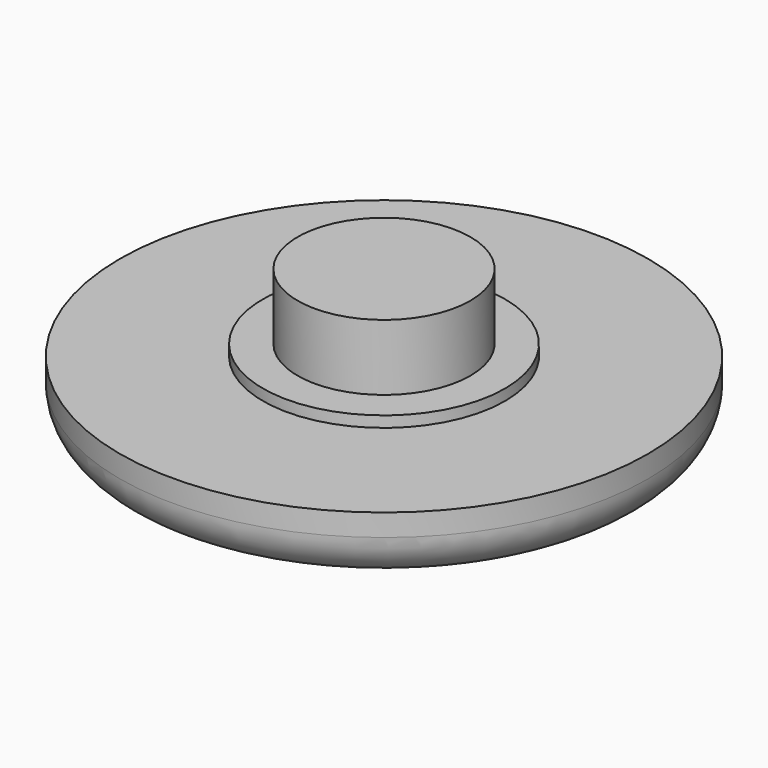
from build123d import *

# Parameters (mm, degrees)
F0_R     = 12
F1_DEPTH = 2
F2_R     = 12
F2_R_2   = 10
F3_DEPTH = 1
F4_R     = 1.99999
F5_R     = 5.5
F6_DEPTH = 0.5
F7_R     = 3.925
F8_DEPTH = 3


# Not quite as in the source:
# - a fillet or chamfer is up to 0.001 mm smaller than in the source, because OpenCascade refuses the exact size


with BuildPart() as f1:
    # F0 (on Top) → F1 (new body)
    with BuildSketch(Plane.XY):
        Circle(F0_R)
    extrude(amount=F1_DEPTH)

    # F2 (on face) → F3 (join)
    with BuildSketch(Plane(origin=(0, 0, 0), x_dir=(1, 0, 0), z_dir=(0, 0, -1))):
        Circle(F2_R)
        Circle(F2_R_2, mode=Mode.SUBTRACT)
    extrude(amount=F3_DEPTH)

    # F4 (radius 2 in the source; OpenCascade refuses exactly that, so slightly less here)
    f4_edges = [f1.edges().sort_by_distance(p)[0] for p in [
        (-12, 0, -1),
    ]]
    fillet(f4_edges, radius=F4_R)

    # F5 (on face) → F6 (join)
    with BuildSketch(Plane.XY.offset(2)):
        Circle(F5_R)
    extrude(amount=F6_DEPTH)

    # F7 (on face) → F8 (join)
    with BuildSketch(Plane.XY.offset(2.5)):
        Circle(F7_R)
    extrude(amount=F8_DEPTH)

    # F9 (on Front) → F10 (revolve)
    with BuildSketch(Plane.XZ):
        Polygon((-10.0021678954, 0), (-10.0021678954, -1.0005384684), (-9.6580199897, -0.9450307698), (-9.385343641, -0.8195927949), (-9.0745007619, -0.6752727786), (-8.19747895, -0.5198512226), (-6.5711033531, -0.3644296667), (-3.5958907101, -0.2090081107), (0, -0.0646880944), (0, 0), align=None)
    revolve(axis=Axis((0, 0, -0.0323440472), (0, 0, 1)))


solid = f1.part
